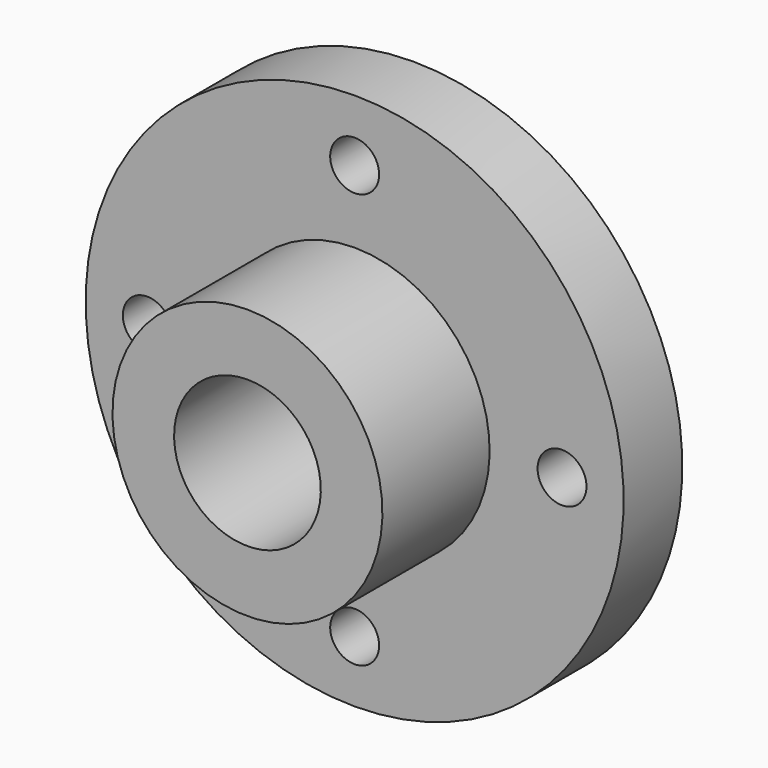
from build123d import *

# Parameters (mm, degrees)
F2_R     = 6.35
F3_DEPTH = 53.849


with BuildPart() as f1:
    # F0 (on Right) → F1 (revolve)
    with BuildSketch(Plane.YZ):
        Polygon((34.798, 35.052), (0, 35.052), (0, 19.05), (53.848, 19.05), (53.848, 69.85), (34.798, 69.85), align=None)
    revolve(axis=Axis((0, 53.1494372582, 0), (0, 1, 0)))

    # F2 (on Front) → F3 (cut, through all)
    with BuildSketch(Plane.XZ):
        with Locations((-53.848, 0)):
            Circle(F2_R)
        with Locations((0, 53.848)):
            Circle(F2_R)
        with Locations((53.848, 0)):
            Circle(F2_R)
        with Locations((0, -53.848)):
            Circle(F2_R)
    extrude(amount=-F3_DEPTH, mode=Mode.SUBTRACT)


solid = f1.part
